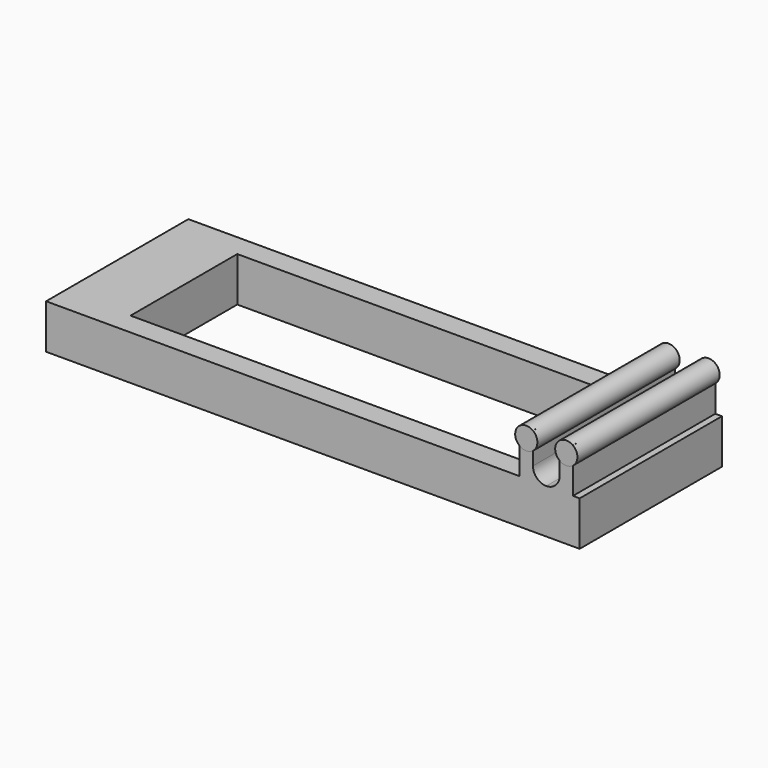
from build123d import *

# Parameters (mm, degrees)
F0_W      = 76.2
F0_H      = 25.4
F0_W_2    = 57.15
F0_H_2    = 19.05
F1_DEPTH  = 6.35
F3_W      = 1.905
F3_H      = 25.4
F4_DEPTH  = 3.81
F5_R      = 1.90499
F6_W      = 1.905
F6_H      = 0.8507965779
F7_DEPTH  = 2.54
F8_R      = 1.5875
F9_DEPTH  = 25.4
F10_W     = 1.905
F10_H     = 0.9408806166
F11_DEPTH = 2.54
F12_R     = 1.5875
F13_DEPTH = 25.4


# Not quite as in the source:
# - a fillet or chamfer is up to 0.001 mm smaller than in the source, because OpenCascade refuses the exact size


with BuildPart() as f1:
    # F0 (on Top) → F1 (new body)
    with BuildSketch(Plane.XY):
        with Locations((27.5905542076, 15.9501524599)):
            Rectangle(F0_W, F0_H)
        with Locations((27.5905542076, 15.9501524599)):
            Rectangle(F0_W_2, F0_H_2, mode=Mode.SUBTRACT)
    extrude(amount=F1_DEPTH)

    # F3 (on face) → F4 (join)
    with BuildSketch(Plane.XY.offset(6.35)):
        with Locations((58.0705542076, 15.9501524599)):
            Rectangle(F3_W, F3_H)
        with Locations((63.7855542076, 15.9501524599)):
            Rectangle(F3_W, F3_H)
    extrude(amount=F4_DEPTH)

    # F5 (radius 1.905 in the source; OpenCascade refuses exactly that, so slightly less here)
    f5_edges = [f1.edges().sort_by_distance(p)[0] for p in [
        (59.023054, 15.950152, 6.35),
        (62.833054, 15.950152, 6.35),
    ]]
    fillet(f5_edges, radius=F5_R)


with BuildPart() as f7:
    # F6 (on face) → F7 (new body)
    with BuildSketch(Plane.XY.offset(10.16)):
        with Locations((63.7855542076, 3.6755507489)):
            Rectangle(F6_W, F6_H)
    extrude(amount=F7_DEPTH)


with BuildPart() as f9:
    # F8 (on face) → F9 (new body, through all)
    with BuildSketch(Plane.XZ.offset(-3.2501524599)):
        with Locations((63.7855542076, 11.43)):
            Circle(F8_R)
    extrude(amount=-F9_DEPTH)


with BuildPart() as f11:
    # F10 (on face) → F11 (new body)
    with BuildSketch(Plane.XY.offset(10.16)):
        with Locations((58.0705542076, 3.7205927682)):
            Rectangle(F10_W, F10_H)
    extrude(amount=F11_DEPTH)


with BuildPart() as f13:
    # F12 (on face) → F13 (new body, through all)
    with BuildSketch(Plane.XZ.offset(-3.2501524599)):
        with Locations((58.0705542076, 11.43)):
            Circle(F12_R)
    extrude(amount=-F13_DEPTH)


solid = Compound([f1.part, f7.part, f9.part, f11.part, f13.part])
